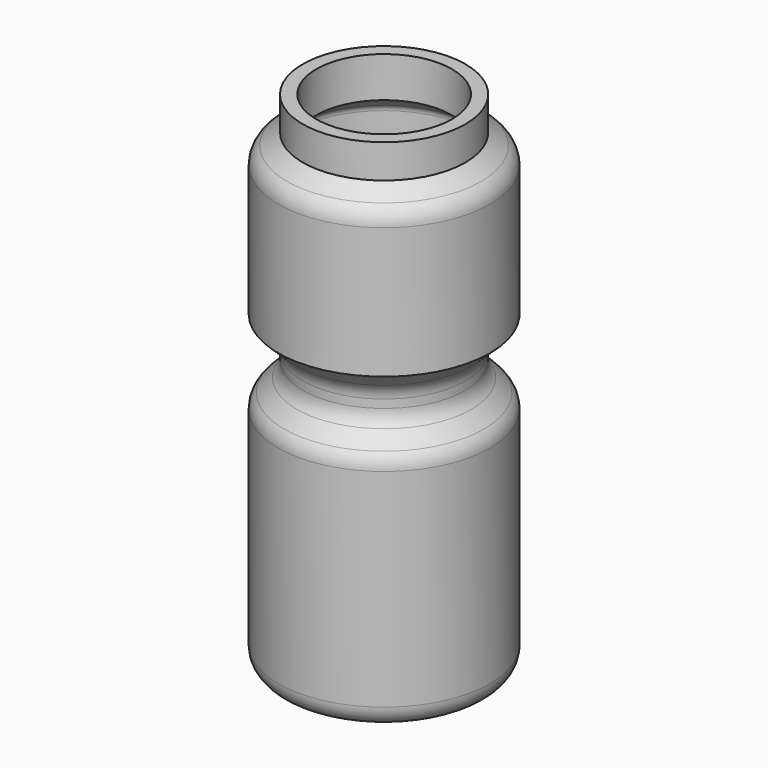
from build123d import *

# Parameters (mm, degrees)
F2_T = -4


with BuildPart() as f1:
    # F0 (on Front) → F1 (revolve)
    with BuildSketch(Plane.XZ):
        with BuildLine():
            Line((0, 150), (0, 0))
            Line((0, 0), (25, 0))
            ThreePointArc((25, 0), (29.4901280605, 1.8598719395), (31.35, 6.35))
            Line((31.35, 6.35), (31.35, 67.835561348))
            ThreePointArc((31.35, 67.835561348), (30.8958269257, 70.1938922964), (29.5982756339, 72.2148719324))
            Line((29.5982756339, 72.2148719324), (25.8603454151, 76.1396982527))
            ThreePointArc((25.8603454151, 76.1396982527), (24.5627941233, 78.1606778887), (24.108621049, 80.5190088371))
            Line((24.108621049, 80.5190088371), (24.108621049, 82.9682330581))
            ThreePointArc((24.108621049, 82.9682330581), (24.6220500432, 85.469620452), (26.0793104646, 87.566508692))
            Line((26.0793104646, 87.566508692), (31.35, 92.5862135351))
            Line((31.35, 92.5862135351), (31.35, 131.4555426863))
            ThreePointArc((31.35, 131.4555426863), (30.6675289492, 134.3193889828), (28.766813981, 136.5676471876))
            Line((28.766813981, 136.5676471876), (24.108621049, 140))
            Line((24.108621049, 140), (24.108621049, 150))
            Line((24.108621049, 150), (0, 150))
        make_face()
    revolve(axis=Axis((0, 0, 75), (0, 0, -1)))

    # F2
    f2_openings = [f1.faces().sort_by_distance(p)[0] for p in [
        (0, 0, 150),
    ]]
    offset(amount=F2_T, openings=f2_openings, kind=Kind.INTERSECTION)


solid = f1.part
